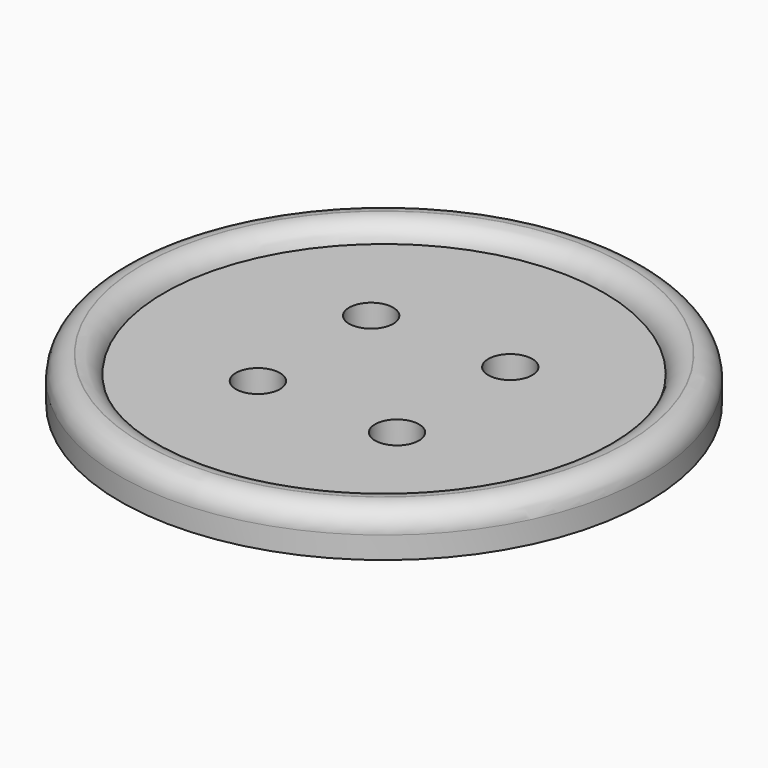
from build123d import *

# Parameters (mm, degrees)
F0_R     = 25
F1_DEPTH = 3
F0_R_2   = 30
F2_DEPTH = 5
F4_R     = 2.5019013152
F5_DEPTH = 25


# Not quite as in the source:
# - a fillet or chamfer that OpenCascade refuses, or shapes differently, is made with other operations: its cross-section is extruded or revolved along the edge and cut away or added


with BuildPart() as f1:
    # F0 (on Top) → F1 (new body)
    with BuildSketch(Plane.XY):
        Circle(F0_R)
    extrude(amount=F1_DEPTH)

    # F0 (on Top) → F2 (join)
    with BuildSketch(Plane.XY):
        Circle(F0_R_2)
        Circle(F0_R, mode=Mode.SUBTRACT)
    extrude(amount=F2_DEPTH)

    # F3: fillet of radius 2.5 on 2 edges, made by hand

    # F3_s1 → F3_t2 (revolve, cut)
    with BuildSketch(Plane.XZ):
        with BuildLine():
            ThreePointArc((30, 2.5), (29.267766953, 4.267766953), (27.5, 5))
            Line((27.5, 5), (30, 5))
            Line((30, 5), (30, 2.5))
        make_face()
    revolve(axis=Axis((0, 0, 5), (0, 0, 1)), mode=Mode.SUBTRACT)

    # F3_s3 → F3_t4 (revolve, cut)
    with BuildSketch(Plane.XZ):
        with BuildLine():
            ThreePointArc((27.4494897428, 5), (25.8683509127, 4.4364916731), (25, 3))
            Line((25, 3), (25, 5))
            Line((25, 5), (27.4494897428, 5))
        make_face()
    revolve(axis=Axis((0, 0, 5), (0, 0, 1)), mode=Mode.SUBTRACT)

    # F4 (on face) → F5 (cut)
    with BuildSketch(Plane.XY.offset(3)):
        with Locations((-7.9056667164, 8.0453660339)):
            Circle(F4_R)
        with Locations((7.9056667164, -8.0453660339)):
            Circle(F4_R)
        with Locations((7.9056667164, 8.0453660339)):
            Circle(F4_R)
        with Locations((-7.9056667164, -8.0453660339)):
            Circle(F4_R)
    extrude(amount=-F5_DEPTH, mode=Mode.SUBTRACT)


solid = f1.part
